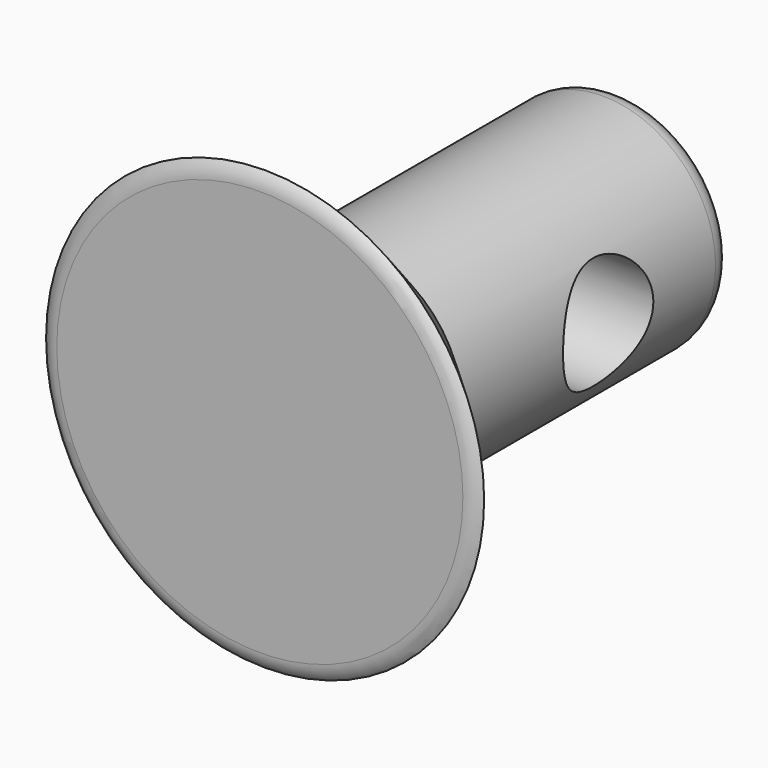
from build123d import *

# Parameters (mm, degrees)
F0_R     = 50.8
F1_DEPTH = 25.4
F2_R     = 5.08
F4_DEPTH = 76.2
F5_R     = 5.08
F7_D     = 25.4
F7_DEPTH = 25.401


# Not quite as in the source:
# - a fillet or chamfer that OpenCascade refuses, or shapes differently, is made with other operations: its cross-section is extruded or revolved along the edge and cut away or added


with BuildPart() as f1:
    # F0 (on Front) → F1 (new body)
    with BuildSketch(Plane.XZ):
        Circle(F0_R)
    extrude(amount=F1_DEPTH)

    # F2
    f2_edges = [f1.edges().sort_by_distance(p)[0] for p in [
        (-50.8, -25.4, 0),
    ]]
    fillet(f2_edges, radius=F2_R)

    # F3: chamfer of 25.4 on 1 edges, made by hand

    # F3_s1 → F3_t2 (revolve, cut)
    with BuildSketch(Plane.XY):
        Polygon((50.8, -25.4), (25.4, 0), (50.8, 0), align=None)
    revolve(axis=Axis((0, 0, 0), (0, -1, 0)), mode=Mode.SUBTRACT)


with BuildPart() as f4:
    # F4 (new): a face of the model
    f4_faces = [f1.part.faces().sort_by_distance(p)[0] for p in [
        (0, 0, 0),
    ]]
    extrude(f4_faces, amount=F4_DEPTH)

    # F5
    f5_edges = [f4.edges().sort_by_distance(p)[0] for p in [
        (-25.4, 76.2, 0),
    ]]
    fillet(f5_edges, radius=F5_R)

    # F7 (through all, one way)
    with BuildSketch(Plane(origin=(0, 0, 0), x_dir=(0, 1, 0), z_dir=(-1, 0, 0))):
        with Locations((40.8925935626, 0)):
            Circle(F7_D / 2)
    extrude(amount=-F7_DEPTH, mode=Mode.SUBTRACT)


solid = Compound([f1.part, f4.part])
